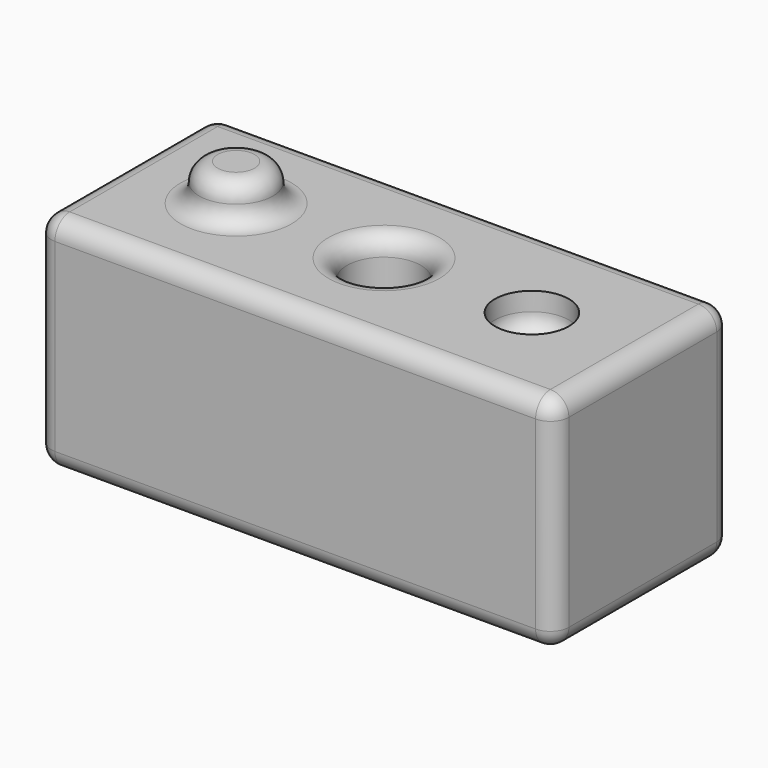
from build123d import *

# Parameters (mm, degrees)
F0_W     = 140
F0_H     = 60
F1_DEPTH = 60
F2_R     = 10
F5_DEPTH = 10
F4_R     = 10
F6_DEPTH = 93.7
F3_R     = 10
F7_DEPTH = 10
F8_R     = 4.99999


# Not quite as in the source:
# - a fillet or chamfer is up to 0.001 mm smaller than in the source, because OpenCascade refuses the exact size


with BuildPart() as f1:
    # F0 (on Top) → F1 (new body)
    with BuildSketch(Plane.XY):
        Rectangle(F0_W, F0_H)
    extrude(amount=F1_DEPTH)

    # F2 (on face) → F5 (join)
    with BuildSketch(Plane.XY.offset(60)):
        with Locations((-40, 0)):
            Circle(F2_R)
    extrude(amount=F5_DEPTH)

    # F4 (on face) → F6 (cut)
    with BuildSketch(Plane.XY.offset(60)):
        Circle(F4_R)
    extrude(amount=-F6_DEPTH, mode=Mode.SUBTRACT)

    # F3 (on face) → F7 (cut)
    with BuildSketch(Plane.XY.offset(60)):
        with Locations((40, 0)):
            Circle(F3_R)
    extrude(amount=-F7_DEPTH, mode=Mode.SUBTRACT)

    # F8 (radius 5 in the source; OpenCascade refuses exactly that, so slightly less here)
    f8_edges = [f1.edges().sort_by_distance(p)[0] for p in [
        (0, 30, 60),
        (70, 0, 60),
        (0, -30, 60),
        (-70, 0, 60),
        (70, -30, 30),
        (70, 30, 30),
        (-70, -30, 30),
        (-70, 30, 30),
        (-50, 0, 70),
        (-10, 0, 60),
        (10, 0, 30),
        (-10, 0, 0),
        (30, 0, 50),
        (-50, 0, 60),
        (0, -30, 0),
        (70, 0, 0),
        (0, 30, 0),
        (-70, 0, 0),
    ]]
    fillet(f8_edges, radius=F8_R)


solid = f1.part
